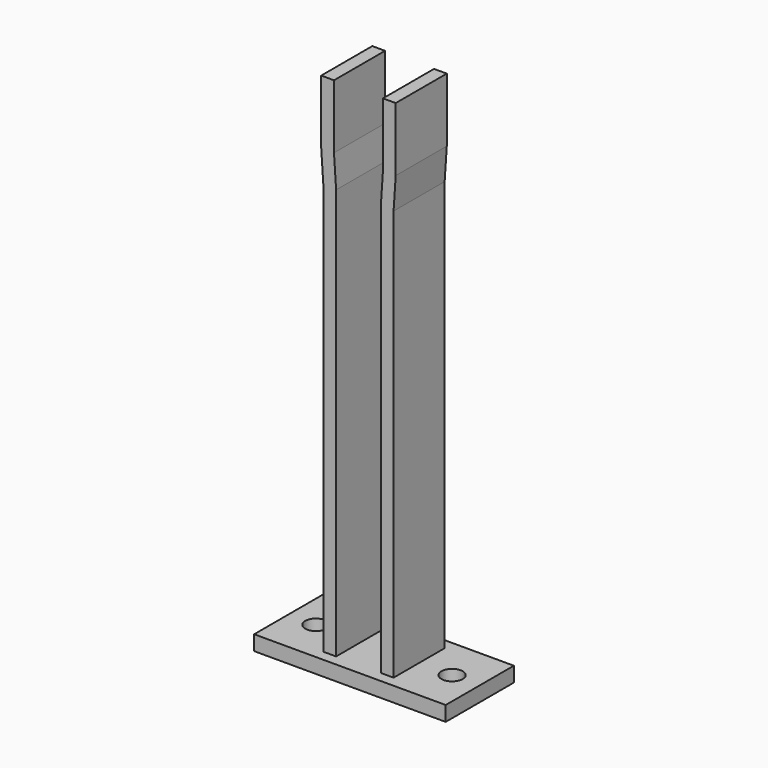
from build123d import *

# Parameters (mm, degrees)
F0_W     = 40
F0_H     = 7
F1_DEPTH = 90
F4_D     = 10
F5_W     = 6
F5_H     = 30
F5_H_2   = 200
F6_DEPTH = 15
F7_DEPTH = 15


# Not quite as in the source:
# - a feature names something its author has since deleted; it is built from what else it names


with BuildPart() as f1:
    # F0 (on Right) → F1 (new body)
    with BuildSketch(Plane.YZ):
        with Locations((0, 3.5)):
            Rectangle(F0_W, F0_H)
    extrude(amount=F1_DEPTH)

    # F4 (through all)
    with Locations(Plane(origin=(0, 0, 0), x_dir=(1, 0, 0), z_dir=(0, 0, -1))):
        with Locations((13, 0), (77, 0)):
            Hole(F4_D / 2)

    # F5 (on Front) → F6 (join)
    with BuildSketch(Plane.XZ):
        with Locations((59.5, 230)):
            Rectangle(F5_W, F5_H)
        Polygon((56.5, 215), (55.5, 200), (61.5, 200), (62.5, 215), align=None)
        with Locations((58.5, 100)):
            Rectangle(F5_W, F5_H_2)
        with Locations((31.5, 100)):
            Rectangle(F5_W, F5_H_2)
        Polygon((27.5, 215), (28.5, 200), (34.5, 200), (33.5, 215), align=None)
        with Locations((30.5, 230)):
            Rectangle(F5_W, F5_H)
    extrude(amount=F6_DEPTH)

    # F7 (add): faces of the model
    f7_faces = [f1.faces().sort_by_distance(p)[0] for p in [
        (31.3424369748, 0, 126),
        (58.6575630252, 0, 126),
    ]]
    extrude(f7_faces, amount=F7_DEPTH)


solid = f1.part
